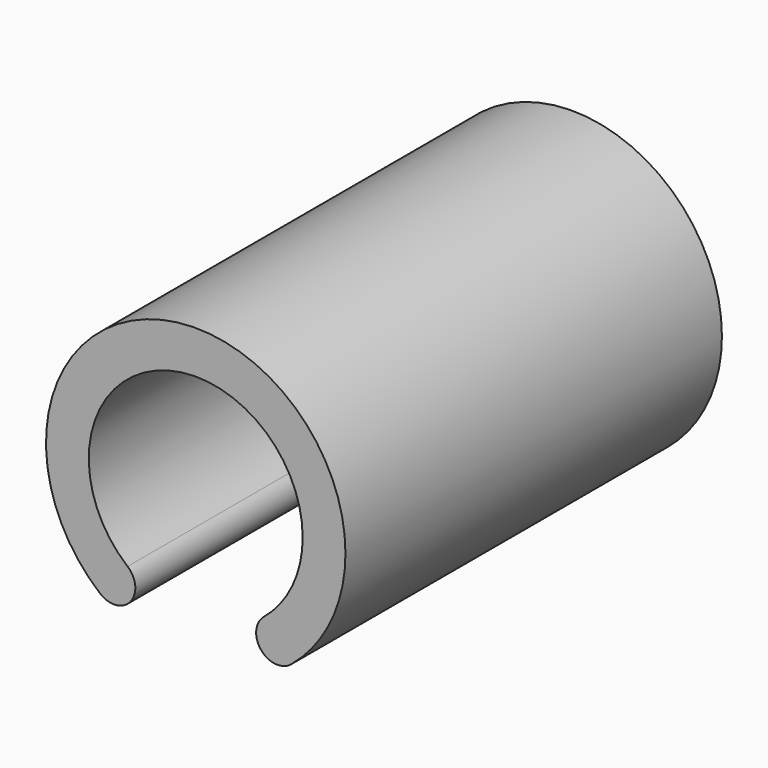
from build123d import *

# Parameters (mm, degrees)
F1_DEPTH = 11
F2_R     = 0.99999


# Not quite as in the source:
# - a fillet or chamfer is up to 0.001 mm smaller than in the source, because OpenCascade refuses the exact size


with BuildPart() as f1:
    # F0 (on Front) → F1 (new body, symmetric)
    with BuildSketch(Plane.XZ):
        with BuildLine():
            Line((-3.5, -6.0621778265), (-2.5, -4.3301270189))
            ThreePointArc((-2.5, -4.3301270189), (-2.5, 4.3301270189), (5, 0))
            ThreePointArc((5, 0), (4.3301270189, -2.5), (2.5, -4.3301270189))
            Line((2.5, -4.3301270189), (3.5, -6.0621778265))
            ThreePointArc((3.5, -6.0621778265), (6.0621778265, -3.5), (7, 0))
            ThreePointArc((7, 0), (-3.5, 6.0621778265), (-3.5, -6.0621778265))
        make_face()
    extrude(amount=F1_DEPTH, both=True)

    # F2 (radius 1 in the source; OpenCascade refuses exactly that, so slightly less here)
    f2_edges = [f1.edges().sort_by_distance(p)[0] for p in [
        (3.5, 5.5, -6.062178),
        (3.5, -5.5, -6.062178),
        (2.5, -5.5, -4.330127),
        (-2.5, -5.5, -4.330127),
        (-3.5, 5.5, -6.062178),
        (-3.5, -5.5, -6.062178),
    ]]
    fillet(f2_edges, radius=F2_R)


solid = f1.part
